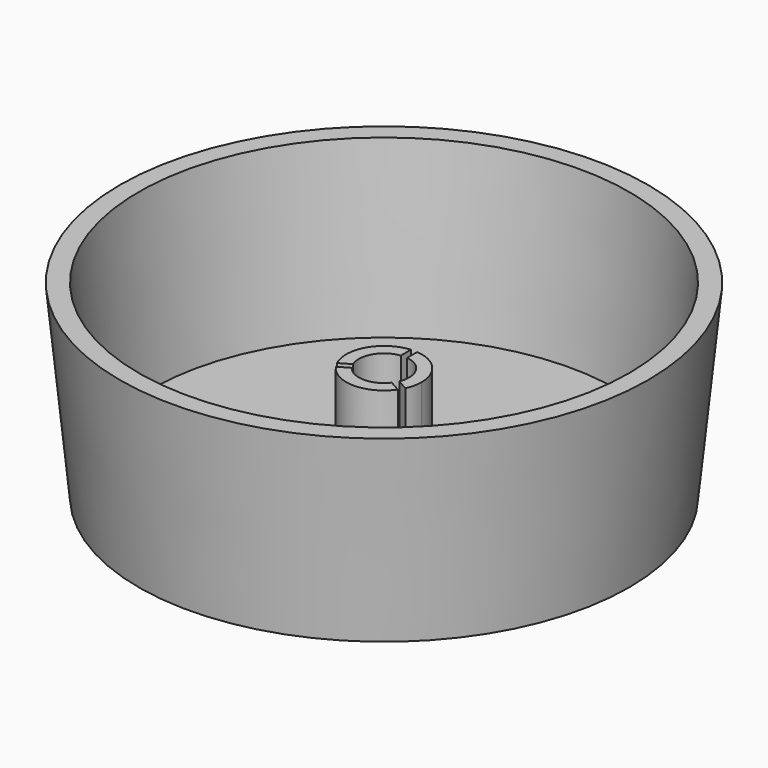
from build123d import *

# Parameters (mm, degrees)
F0_R     = 21
F1_DEPTH = 15
F2_DEPTH = 1.5
F3_DEPTH = 1
F4_DEPTH = 9
F5_SIZE2 = 1.49999
F5_SIZE  = 14.99999


# Not quite as in the source:
# - a fillet or chamfer that OpenCascade refuses, or shapes differently, is made with other operations: its cross-section is extruded or revolved along the edge and cut away or added
# - a fillet or chamfer is up to 0.001 mm smaller than in the source, because OpenCascade refuses the exact size


with BuildPart() as f1:
    # F0 (on Top) → F1 (new body)
    with BuildSketch(Plane.XY):
        Circle(F0_R)
        with BuildLine():
            ThreePointArc((0.5, 18.4932420089), (13.2570735836, 12.9034879006), (18.5, 0))
            ThreePointArc((18.5, 0), (-12.9034879006, -13.2570735836), (-0.5, 18.4932420089))
            ThreePointArc((-0.5, 18.4932420089), (0, 18.5), (0.5, 18.4932420089))
        make_face(mode=Mode.SUBTRACT)
    extrude(amount=F1_DEPTH)

    # F0 (on Top) → F2 (join)
    with BuildSketch(Plane.XY):
        with BuildLine():
            ThreePointArc((-0.5, 18.4932420089), (-12.9034879006, -13.2570735836), (18.5, 0))
            ThreePointArc((18.5, 0), (13.2570735836, 12.9034879006), (0.5, 18.4932420089))
            Line((0.5, 18.4932420089), (0.5, 8.4932420089))
            ThreePointArc((0.5, 8.4932420089), (0, 7.9932420089), (-0.5, 8.4932420089))
            Line((-0.5, 8.4932420089), (-0.5, 18.4932420089))
        make_face()
        with BuildLine():
            ThreePointArc((0.25, 2.9895651858), (2.2079402166, 2.0310096012), (3, 0))
            ThreePointArc((3, 0), (2.9276371182, -0.6549358016), (2.7140393972, -1.2782762419))
            ThreePointArc((2.7140393972, -1.2782762419), (2.5980762114, -1.5), (2.4640393972, -1.7112889438))
            ThreePointArc((2.4640393972, -1.7112889438), (0, -3), (-2.4640393972, -1.7112889438))
            ThreePointArc((-2.4640393972, -1.7112889438), (-2.5980762114, -1.5), (-2.7140393972, -1.2782762419))
            ThreePointArc((-2.7140393972, -1.2782762419), (-2.5980762114, 1.5), (-0.25, 2.9895651858))
            ThreePointArc((-0.25, 2.9895651858), (0, 3), (0.25, 2.9895651858))
        make_face(mode=Mode.SUBTRACT)
        with BuildLine():
            ThreePointArc((2, 0), (1.5, 1.3228756555), (0.25, 1.9843134833))
            ThreePointArc((0.25, 1.9843134833), (0, 2), (-0.25, 1.9843134833))
            ThreePointArc((-0.25, 1.9843134833), (-1.7320508076, 1), (-1.8434658856, -0.7756503907))
            ThreePointArc((-1.8434658856, -0.7756503907), (-1.7320508076, -1), (-1.5934658856, -1.2086630926))
            ThreePointArc((-1.5934658856, -1.2086630926), (0, -2), (1.5934658856, -1.2086630926))
            ThreePointArc((1.5934658856, -1.2086630926), (1.7320508076, -1), (1.8434658856, -0.7756503907))
            ThreePointArc((1.8434658856, -0.7756503907), (1.9604759334, -0.3956439237), (2, 0))
        make_face()
        with BuildLine():
            Line((0.5, 8.4932420089), (0.5, 18.4932420089))
            Line((0.5, 18.4932420089), (-0.5, 18.4932420089))
            Line((-0.5, 18.4932420089), (-0.5, 8.4932420089))
            ThreePointArc((-0.5, 8.4932420089), (0, 8.9932420089), (0.5, 8.4932420089))
        make_face()
        with BuildLine():
            Line((-0.25, 1.9843134833), (-0.25, 2.9895651858))
            ThreePointArc((-0.25, 2.9895651858), (-2.5980762114, 1.5), (-2.7140393972, -1.2782762419))
            Line((-2.7140393972, -1.2782762419), (-1.8434658856, -0.7756503907))
            ThreePointArc((-1.8434658856, -0.7756503907), (-1.7320508076, 1), (-0.25, 1.9843134833))
        make_face()
        with BuildLine():
            ThreePointArc((-2.4640393972, -1.7112889438), (0, -3), (2.4640393972, -1.7112889438))
            Line((2.4640393972, -1.7112889438), (1.5934658856, -1.2086630926))
            ThreePointArc((1.5934658856, -1.2086630926), (0, -2), (-1.5934658856, -1.2086630926))
            Line((-1.5934658856, -1.2086630926), (-2.4640393972, -1.7112889438))
        make_face()
        with BuildLine():
            ThreePointArc((2.7140393972, -1.2782762419), (2.9276371182, -0.6549358016), (3, 0))
            ThreePointArc((3, 0), (2.2079402166, 2.0310096012), (0.25, 2.9895651858))
            Line((0.25, 2.9895651858), (0.25, 1.9843134833))
            ThreePointArc((0.25, 1.9843134833), (1.5, 1.3228756555), (2, 0))
            ThreePointArc((2, 0), (1.9604759334, -0.3956439237), (1.8434658856, -0.7756503907))
            Line((1.8434658856, -0.7756503907), (2.7140393972, -1.2782762419))
        make_face()
        with BuildLine():
            Line((0.25, 1.9843134833), (0.25, 2.9895651858))
            ThreePointArc((0.25, 2.9895651858), (0, 3), (-0.25, 2.9895651858))
            Line((-0.25, 2.9895651858), (-0.25, 1.9843134833))
            ThreePointArc((-0.25, 1.9843134833), (0, 2), (0.25, 1.9843134833))
        make_face()
        with BuildLine():
            ThreePointArc((2.4640393972, -1.7112889438), (2.5980762114, -1.5), (2.7140393972, -1.2782762419))
            Line((2.7140393972, -1.2782762419), (1.8434658856, -0.7756503907))
            ThreePointArc((1.8434658856, -0.7756503907), (1.7320508076, -1), (1.5934658856, -1.2086630926))
            Line((1.5934658856, -1.2086630926), (2.4640393972, -1.7112889438))
        make_face()
        with BuildLine():
            Line((-1.8434658856, -0.7756503907), (-2.7140393972, -1.2782762419))
            ThreePointArc((-2.7140393972, -1.2782762419), (-2.5980762114, -1.5), (-2.4640393972, -1.7112889438))
            Line((-2.4640393972, -1.7112889438), (-1.5934658856, -1.2086630926))
            ThreePointArc((-1.5934658856, -1.2086630926), (-1.7320508076, -1), (-1.8434658856, -0.7756503907))
        make_face()
        with BuildLine():
            ThreePointArc((-0.5, 8.4932420089), (0, 7.9932420089), (0.5, 8.4932420089))
            Line((0.5, 8.4932420089), (-0.5, 8.4932420089))
        make_face()
        with BuildLine():
            Line((-0.5, 8.4932420089), (0.5, 8.4932420089))
            ThreePointArc((0.5, 8.4932420089), (0, 8.9932420089), (-0.5, 8.4932420089))
        make_face()
        with BuildLine():
            Line((-0.5, 18.4932420089), (0.5, 18.4932420089))
            ThreePointArc((0.5, 18.4932420089), (0, 18.5), (-0.5, 18.4932420089))
        make_face()
    extrude(amount=F2_DEPTH)

    # F0 (on Top) → F3 (cut)
    with BuildSketch(Plane.XY):
        with BuildLine():
            ThreePointArc((-0.5, 8.4932420089), (0, 7.9932420089), (0.5, 8.4932420089))
            Line((0.5, 8.4932420089), (-0.5, 8.4932420089))
        make_face()
        with BuildLine():
            Line((-0.5, 8.4932420089), (0.5, 8.4932420089))
            ThreePointArc((0.5, 8.4932420089), (0, 8.9932420089), (-0.5, 8.4932420089))
        make_face()
        with BuildLine():
            Line((-0.5, 18.4932420089), (0.5, 18.4932420089))
            ThreePointArc((0.5, 18.4932420089), (0, 18.5), (-0.5, 18.4932420089))
        make_face()
        with BuildLine():
            Line((0.5, 8.4932420089), (0.5, 18.4932420089))
            Line((0.5, 18.4932420089), (-0.5, 18.4932420089))
            Line((-0.5, 18.4932420089), (-0.5, 8.4932420089))
            ThreePointArc((-0.5, 8.4932420089), (0, 8.9932420089), (0.5, 8.4932420089))
        make_face()
    extrude(amount=F3_DEPTH, mode=Mode.SUBTRACT)

    # F0 (on Top) → F4 (join)
    with BuildSketch(Plane.XY):
        with BuildLine():
            Line((-0.25, 1.9843134833), (-0.25, 2.9895651858))
            ThreePointArc((-0.25, 2.9895651858), (-2.5980762114, 1.5), (-2.7140393972, -1.2782762419))
            Line((-2.7140393972, -1.2782762419), (-1.8434658856, -0.7756503907))
            ThreePointArc((-1.8434658856, -0.7756503907), (-1.7320508076, 1), (-0.25, 1.9843134833))
        make_face()
        with BuildLine():
            ThreePointArc((2.7140393972, -1.2782762419), (2.9276371182, -0.6549358016), (3, 0))
            ThreePointArc((3, 0), (2.2079402166, 2.0310096012), (0.25, 2.9895651858))
            Line((0.25, 2.9895651858), (0.25, 1.9843134833))
            ThreePointArc((0.25, 1.9843134833), (1.5, 1.3228756555), (2, 0))
            ThreePointArc((2, 0), (1.9604759334, -0.3956439237), (1.8434658856, -0.7756503907))
            Line((1.8434658856, -0.7756503907), (2.7140393972, -1.2782762419))
        make_face()
        with BuildLine():
            ThreePointArc((-2.4640393972, -1.7112889438), (0, -3), (2.4640393972, -1.7112889438))
            Line((2.4640393972, -1.7112889438), (1.5934658856, -1.2086630926))
            ThreePointArc((1.5934658856, -1.2086630926), (0, -2), (-1.5934658856, -1.2086630926))
            Line((-1.5934658856, -1.2086630926), (-2.4640393972, -1.7112889438))
        make_face()
    extrude(amount=F4_DEPTH)

    # F5 (size 15 and 1.5 in the source; OpenCascade refuses exactly that, so slightly less here)
    f5_edges = [f1.edges().sort_by_distance(p)[0] for p in [
        (-21, 0, 0),
    ]]
    f5_side = f1.faces().sort_by_distance((-21, 0, 7.5))[0]
    chamfer(f5_edges, length=F5_SIZE, length2=F5_SIZE2, reference=f5_side)

    # F6: chamfer of 14 x 1 on 1 edges, made by hand


with BuildPart() as f6_tool2:
    # F6_s3 → F6_t4 (revolve)
    with BuildSketch(Plane(origin=(0, 0, 0), x_dir=(0, 0, 1), z_dir=(0.9996347032, 0.027027027, 0))):
        Polygon((15, -19.5), (1, -18.5), (15, -18.5), align=None)
    revolve(axis=Axis((0, 0, 15), (0, 0, 1)))

    split(bisect_by=Plane.XY.offset(1.5), keep=Keep.TOP)


with BuildPart() as f1_1:
    add(f1.part)

    # F6_t1: cut F6_tool2
    add(f6_tool2.part, mode=Mode.SUBTRACT)


solid = f1_1.part
